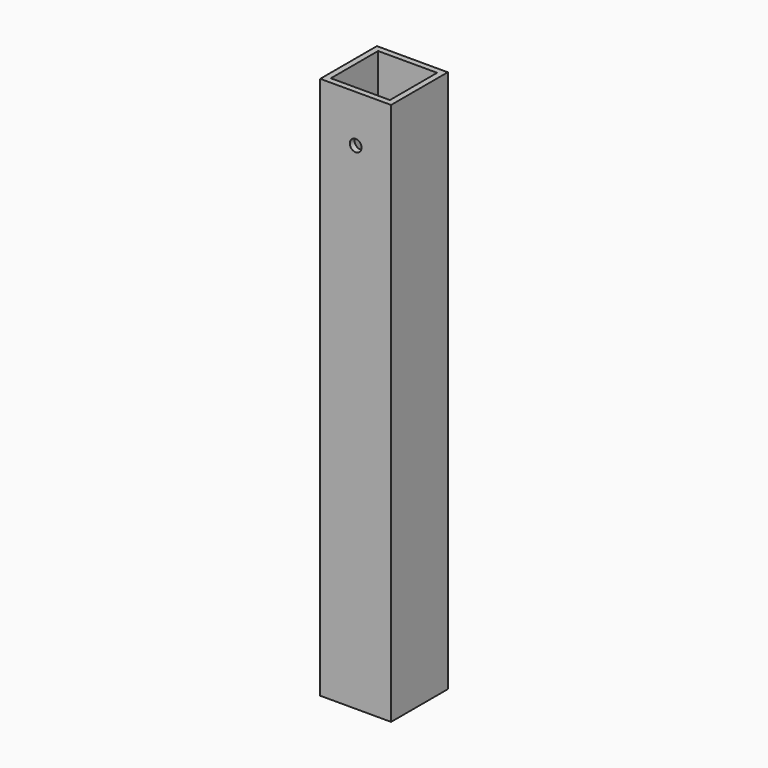
from build123d import *

# Parameters (mm, degrees)
F0_W     = 76.2
F0_H     = 76.2
F0_W_2   = 63.5
F0_H_2   = 63.5
F1_DEPTH = 584.2
F3_D     = 12.7


# Not quite as in the source:
# - a length typed as a fraction of an inch, garbled in the dataset ("3 / 203.2 mm" for 3/8 in), is restored


with BuildPart() as f1:
    # F0 (on Top) → F1 (new body)
    with BuildSketch(Plane.XY):
        Rectangle(F0_W, F0_H)
        Rectangle(F0_W_2, F0_H_2, mode=Mode.SUBTRACT)
    extrude(amount=F1_DEPTH)

    # F3 (through all)
    with Locations(Plane.XZ.offset(38.1)):
        with Locations((0, 533.4)):
            Hole(F3_D / 2)


solid = f1.part
